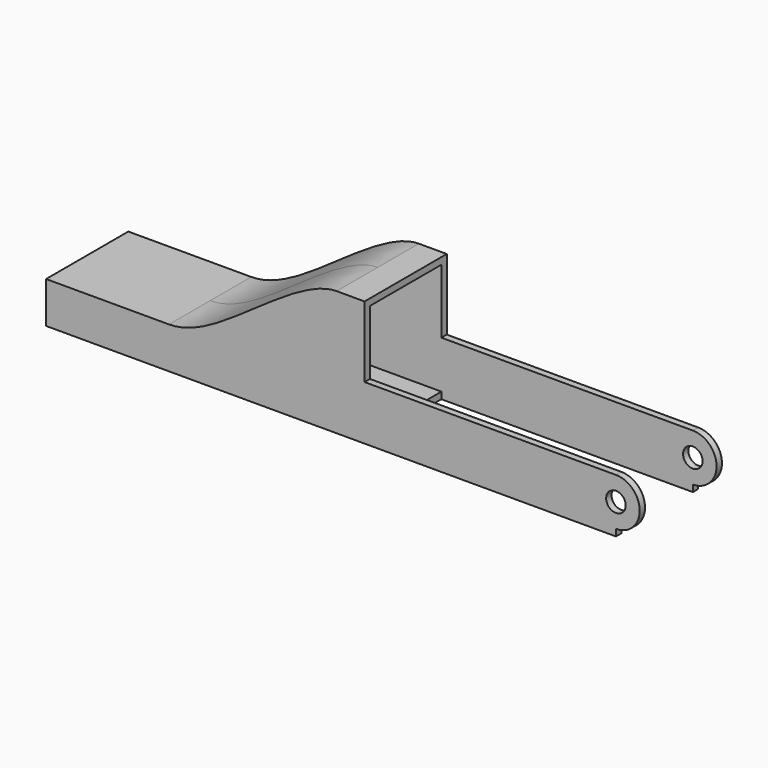
from build123d import *

# Parameters (mm, degrees)
F0_W     = 45
F0_H     = 8.5
F0_H_2   = 1.2
F0_W_2   = 22
F0_H_3   = 5
F1_DEPTH = 1.2
F2_DEPTH = 9.2
F3_D     = 3.5


# Not quite as in the source:
# - the dataset's text gives a spline's control points without its knots; the knots are read off the source's solid


with BuildPart() as f1:
    # F0 (on Front) → F1 (new body)
    with BuildSketch(Plane.XZ):
        with BuildLine():
            Line((47.5, -1.5), (47.5, -10))
            ThreePointArc((47.5, -10), (51.75, -5.75), (47.5, -1.5))
        make_face()
        with Locations((25, -5.75)):
            Rectangle(F0_W, F0_H)
        with Locations((25, -10.6)):
            Rectangle(F0_W, F0_H_2)
        with BuildLine():
            Line((-32.5, -10), (-2.5, -10))
            Line((-2.5, -10), (-2.5, 10))
            add(Edge.make_bspline(
                [(-32.5, -5), (-27.5803674012, -5), (-17.2100449751, 2.2275754238), (-6.0579581186, 10), (-2.5, 10)],
                knots=[0, 0, 0, 0, 0.5090778259, 1, 1, 1, 1], degree=3))
            Line((-32.5, -5), (-32.5, -10))
        make_face()
        Polygon((-2.5, -10), (2.5, -10), (2.5, -1.5), (2.5, 10), (-2.5, 10), align=None)
        with Locations((-43.5, -7.5)):
            Rectangle(F0_W_2, F0_H_3)
    extrude(amount=F1_DEPTH)

    # F0 (on Front) → F2 (join)
    with BuildSketch(Plane.XZ):
        with BuildLine():
            add(Edge.make_bspline(
                [(-32.5, -5), (-27.5803674012, -5), (-17.2100449751, 2.2275754238), (-6.0579581186, 10), (-2.5, 10)],
                knots=[0, 0, 0, 0, 0.5090778259, 1, 1, 1, 1], degree=3))
            Line((-2.5, 10), (2.5, 10))
            Line((2.5, 10), (2.5, 11.2))
            Line((2.5, 11.2), (-2.5, 11.2))
            add(Edge.make_bspline(
                [(-32.5, -3.8), (-31.4389363622, -3.8), (-29.2200835852, -3.4091842374), (-25.6037921172, -1.8183804645), (-21.7862624056, 0.5093473763), (-17.819156486, 3.2622809958), (-13.7265020427, 6.1236212623), (-10.3779360475, 8.2729183736), (-7.8194468713, 9.6607467479), (-5.973100675, 10.4877178879), (-4.2025331466, 11.0487112992), (-3.0621946213, 11.2), (-2.5, 11.2)],
                knots=[0, 0, 0, 0, 0.125, 0.25, 0.375, 0.5, 0.625, 0.75, 0.8125, 0.875, 0.9375, 1, 1, 1, 1], degree=3))
            Line((-32.5, -3.8), (-54.5, -3.8))
            Line((-54.5, -3.8), (-54.5, -5))
            Line((-54.5, -5), (-32.5, -5))
        make_face()
        Polygon((2.5, -11.2), (2.5, -10), (-2.5, -10), (-32.5, -10), (-54.5, -10), (-54.5, -11.2), (-32.8350449828, -11.2), (-2.8350449828, -11.2), align=None)
    extrude(amount=F2_DEPTH)

    # F3 (through all)
    with Locations(Plane(origin=(0, 0, 0), x_dir=(1, 0, 0), z_dir=(0, 1, 0))):
        with Locations((47.5, 5.75)):
            Hole(F3_D / 2)

    # F4: F1 across face


with BuildPart() as f1_1:
    add(f1.part)
    add(f1.part.mirror(Plane(origin=(-26, -9.2, -10.6), x_dir=(1, 0, 0), z_dir=(0, -1, 0))))


solid = f1_1.part
